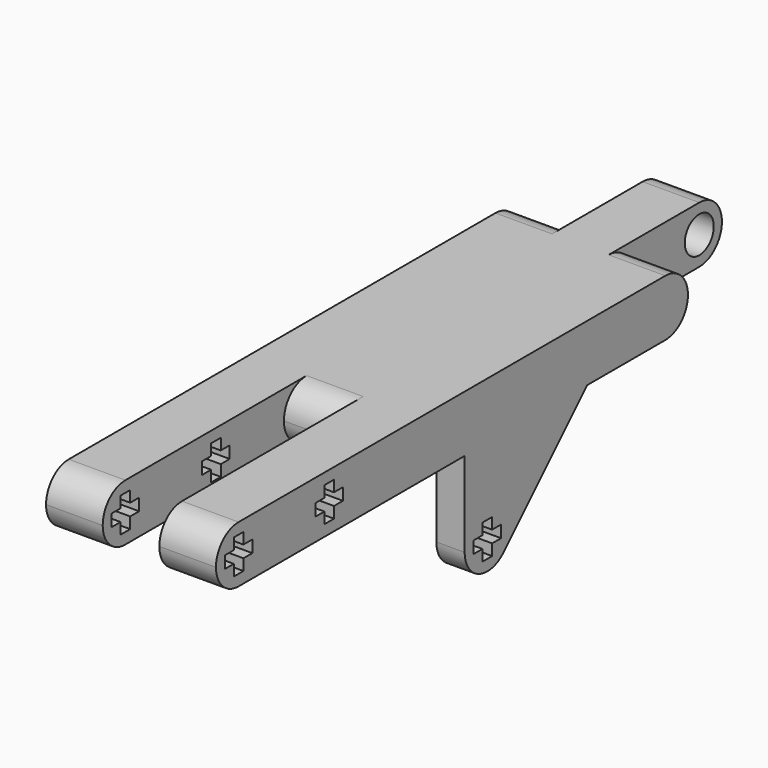
from build123d import *

# Parameters (mm, degrees)
F1_DEPTH  = 7.9375
F2_W      = 3.96875
F2_H      = 7.9375
F3_DEPTH  = 15.875
F4_R      = 3.96874
F5_W      = 1.56845
F5_H      = 1.6891
F5_W_2    = 1.6891
F5_H_2    = 1.56845
F5_R      = 2.54
F6_DEPTH  = 23.8125
F8_DEPTH  = 3.96875
F10_DEPTH = 3.96875


# Not quite as in the source:
# - a fillet or chamfer is up to 0.001 mm smaller than in the source, because OpenCascade refuses the exact size


with BuildPart() as f1:
    # F0 (on Top) → F1 (new body)
    with BuildSketch(Plane.XY):
        Polygon((0, 82.7019174), (0, 0), (7.9375, 0), (7.9375, 31.75), (15.875, 31.75), (15.875, 0), (23.8125, 0), (23.8125, 82.7019174), (15.875, 82.7019174), (15.875, 98.5769174), (7.9375, 98.5769174), (7.9375, 82.7019174), align=None)
    extrude(amount=F1_DEPTH)

    # F2 (on face) → F3 (join)
    with BuildSketch(Plane(origin=(0, 0, 0), x_dir=(1, 0, 0), z_dir=(0, 0, -1))):
        with Locations((21.828125, -47.5457774)):
            Rectangle(F2_W, F2_H)
        with Locations((1.984375, -47.5457774)):
            Rectangle(F2_W, F2_H)
    extrude(amount=F3_DEPTH)

    # F4 (radius 3.96875 in the source; OpenCascade refuses exactly that, so slightly less here)
    f4_edges = [f1.edges().sort_by_distance(p)[0] for p in [
        (19.84375, 82.701917, 0),
        (19.84375, 82.701917, 7.9375),
        (11.90625, 98.576917, 0),
        (11.90625, 98.576917, 7.9375),
        (3.96875, 82.701917, 0),
        (3.96875, 82.701917, 7.9375),
        (1.984375, 51.514527, -15.875),
        (1.984375, 43.577027, -15.875),
        (21.828125, 51.514527, -15.875),
        (21.828125, 43.577027, -15.875),
        (3.96875, 0, 0),
        (3.96875, 0, 7.9375),
        (19.84375, 0, 7.9375),
        (19.84375, 0, 0),
        (11.90625, 31.75, 7.9375),
        (11.90625, 31.75, 0),
    ]]
    fillet(f4_edges, radius=F4_R)

    # F5 (on face) → F6 (cut, through all)
    with BuildSketch(Plane(origin=(0, 0, 0), x_dir=(0, -1, 0), z_dir=(-1, 0, 0))):
        with Locations((-2.339975, 3.96875)):
            Rectangle(F5_W, F5_H)
        with Locations((-3.96875, 2.339975)):
            Rectangle(F5_W_2, F5_H_2)
        with Locations((-3.96875, 3.96875)):
            Rectangle(F5_W_2, F5_H)
        with Locations((-5.597525, 3.96875)):
            Rectangle(F5_W, F5_H)
        with Locations((-3.96875, 5.597525)):
            Rectangle(F5_W_2, F5_H_2)
        with Locations((-47.5457774, -10.277475)):
            Rectangle(F5_W_2, F5_H_2)
        with Locations((-47.5457774, -11.90625)):
            Rectangle(F5_W_2, F5_H)
        with Locations((-49.1745524, -11.90625)):
            Rectangle(F5_W, F5_H)
        with Locations((-45.9170024, -11.90625)):
            Rectangle(F5_W, F5_H)
        with Locations((-47.5457774, -13.535025)):
            Rectangle(F5_W_2, F5_H_2)
        with Locations((-19.84375, 2.339975)):
            Rectangle(F5_W_2, F5_H_2)
        with Locations((-21.472525, 3.96875)):
            Rectangle(F5_W, F5_H)
        with Locations((-19.84375, 3.96875)):
            Rectangle(F5_W_2, F5_H)
        with Locations((-18.214975, 3.96875)):
            Rectangle(F5_W, F5_H)
        with Locations((-19.84375, 5.597525)):
            Rectangle(F5_W_2, F5_H_2)
        with Locations((-94.6081674, 3.96875)):
            Circle(F5_R)
    extrude(amount=-F6_DEPTH, mode=Mode.SUBTRACT)

    # F7 (on face) → F8 (join, through all)
    with BuildSketch(Plane(origin=(0, 0, 0), x_dir=(0, -1, 0), z_dir=(-1, 0, 0))):
        with BuildLine():
            Line((-65.0646874757, 0), (-50.3521074378, -14.7125800378))
            ThreePointArc((-50.3521074378, -14.7125800378), (-51.2124242947, -13.4250248722), (-51.5145274, -11.90625))
            Line((-51.5145274, -11.90625), (-51.5145274, 0))
            Line((-51.5145274, 0), (-65.0646874757, 0))
        make_face()
    extrude(amount=-F8_DEPTH)

    # F9 (on face) → F10 (join, through all)
    with BuildSketch(Plane.YZ.offset(23.8125)):
        with BuildLine():
            ThreePointArc((51.5145274, -11.90625), (51.2124242947, -13.4250248722), (50.3521074378, -14.7125800378))
            Line((50.3521074378, -14.7125800378), (65.0646874757, 0))
            Line((65.0646874757, 0), (51.5145274, 0))
            Line((51.5145274, 0), (51.5145274, -11.90625))
        make_face()
    extrude(amount=-F10_DEPTH)


solid = f1.part
